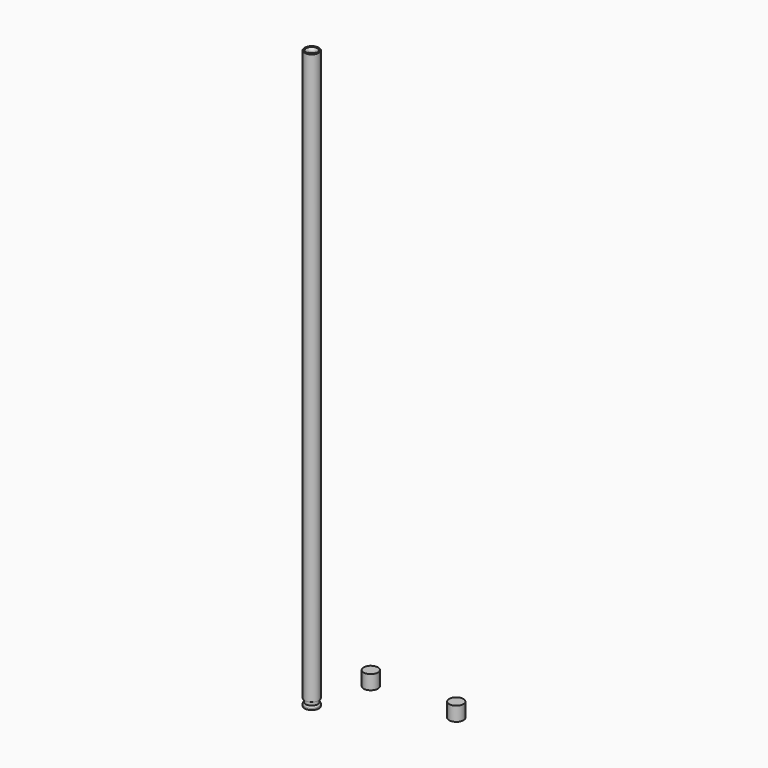
from build123d import *

# Parameters (mm, degrees)
F0_R      = 12.7
F0_R_2    = 11.1125
F1_DEPTH  = 1016
F2_DEPTH  = 6.35
F3_R      = 12.7
F4_DEPTH  = 6.35
F6_R      = 11.1123873654
F6_R_2    = 4.7623887658
F7_DEPTH  = 25.4
F8_DEPTH  = 25.4
F9_SIZE   = 1.27
F10_R     = 5.07999
F12_R     = 12.7
F13_DEPTH = 25.4


# Not quite as in the source:
# - a fillet or chamfer that OpenCascade refuses, or shapes differently, is made with other operations: its cross-section is extruded or revolved along the edge and cut away or added
# - a fillet or chamfer is up to 0.001 mm smaller than in the source, because OpenCascade refuses the exact size


with BuildPart() as f1:
    # F0 (on Top) → F1 (new body)
    with BuildSketch(Plane.XY):
        with Locations((-52.5920726359, -16.7048629373)):
            Circle(F0_R)
        with Locations((-52.5920726359, -16.7048629373)):
            Circle(F0_R_2, mode=Mode.SUBTRACT)
    extrude(amount=F1_DEPTH)

    # F0 (on Top) → F2 (join)
    with BuildSketch(Plane.XY):
        with Locations((-52.5920726359, -16.7048629373)):
            Circle(F0_R_2)
    extrude(amount=-F2_DEPTH)

    # F3 (on face) → F4 (join)
    with BuildSketch(Plane(origin=(0, 0, -6.35), x_dir=(1, 0, 0), z_dir=(0, 0, -1))):
        with Locations((-52.5920726359, 16.7048629373)):
            Circle(F3_R)
    extrude(amount=F4_DEPTH)

    # F5: fillet of radius 5.08 on 1 edges, made by hand

    # F5_s1 → F5_t2 (revolve, cut)
    with BuildSketch(Plane.XZ.offset(16.7048629373)):
        with BuildLine():
            ThreePointArc((-39.8920726359, -10.0390166373), (-40.3057946759, -8.0309703231), (-41.4795726359, -6.35))
            Line((-41.4795726359, -6.35), (-41.4097226359, -6.2762196673))
            ThreePointArc((-41.4097226359, -6.2762196673), (-40.6858226359, -6.2484), (-39.8920726359, -6.2484))
            Line((-39.8920726359, -6.2484), (-39.7904726359, -6.35))
            Line((-39.7904726359, -6.35), (-39.7904726359, -10.0390166373))
            Line((-39.7904726359, -10.0390166373), (-39.8920726359, -10.0390166373))
        make_face()
    revolve(axis=Axis((-52.5920726359, -16.7048629373, -6.35), (0, 0, -1)), mode=Mode.SUBTRACT)


with BuildPart() as f7:
    # F6 (on face) → F7 (new body)
    with BuildSketch(Plane.XY.offset(1016)):
        with Locations((-52.5920726359, -16.7048629373)):
            Circle(F6_R)
        with Locations((-52.5920726359, -16.7048629373)):
            Circle(F6_R_2, mode=Mode.SUBTRACT)
    extrude(amount=-F7_DEPTH)

    # F6 (on face) → F8 (join)
    with BuildSketch(Plane.XY.offset(1016)):
        with Locations((-52.5920726359, -16.7048629373)):
            Circle(F6_R)
        with Locations((-52.5920726359, -16.7048629373)):
            Circle(F6_R_2, mode=Mode.SUBTRACT)
    extrude(amount=-F8_DEPTH)

    # F9
    f9_edges = [f7.edges().sort_by_distance(p)[0] for p in [
        (-63.70446, -16.704863, 1016),
    ]]
    chamfer(f9_edges, length=F9_SIZE)

    # F10 (radius 5.08 in the source; OpenCascade refuses exactly that, so slightly less here)
    f10_edges = [f7.edges().sort_by_distance(p)[0] for p in [
        (-57.354461, -16.704863, 1016),
    ]]
    fillet(f10_edges, radius=F10_R)


with BuildPart() as f13:
    # F12 (on Top) → F13 (new body)
    with BuildSketch(Plane.XY):
        with Locations((-10.5100030951, 62.1974789812)):
            Circle(F12_R)
    extrude(amount=F13_DEPTH)


with BuildPart() as f13b:
    # F12 (on Top) → F13, piece 2 (new body)
    with BuildSketch(Plane.XY):
        with Locations((141.8899969049, 62.1974789812)):
            Circle(F12_R)
    extrude(amount=F13_DEPTH)


with BuildPart() as f1_1:
    # F14: moved
    add(f1.part)


solid = Compound([f7.part, f13.part, f13b.part, f1_1.part])
